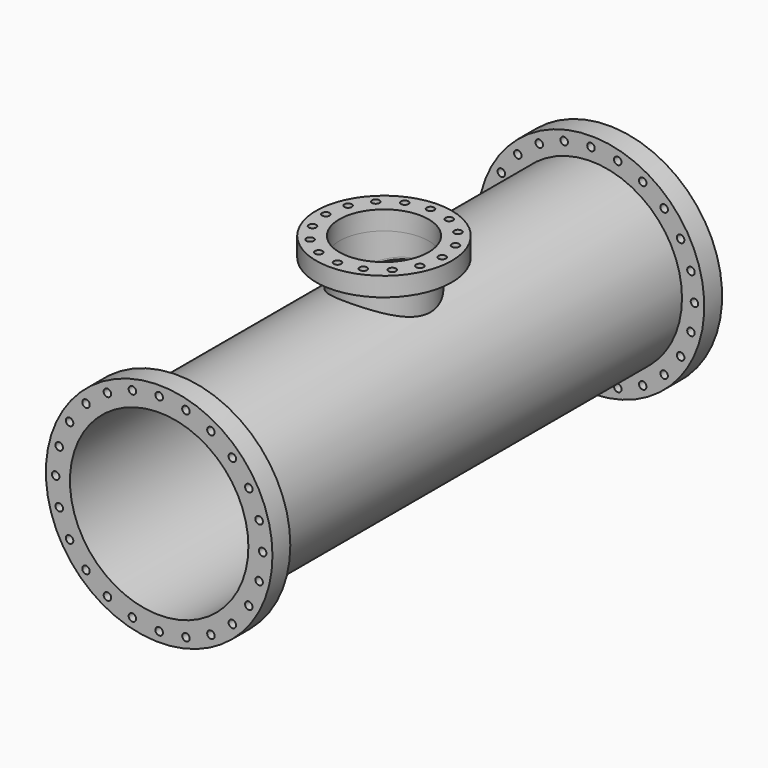
from build123d import *

# Parameters (mm, degrees)
F0_R      = 102
F0_R_2    = 100
F1_DEPTH  = 580
F2_R      = 127
F2_R_2    = 102
F2_R_3    = 100
F3_DEPTH  = 25
F4_R      = 127
F4_R_2    = 102
F4_R_3    = 100
F5_DEPTH  = 25
F7_D      = 8.4
F9_R      = 52
F9_R_2    = 50
F10_REACH = 399.0792104868
F11_REACH = 393.4223562373
F9_R_3    = 76
F12_DEPTH = 21.3
F14_D     = 8.4
F14_DEPTH = 27
F14_TIP   = 2.5236145999


with BuildPart() as f1:
    # F0 (on Front) → F1 (new body)
    with BuildSketch(Plane.XZ):
        Circle(F0_R)
        Circle(F0_R_2, mode=Mode.SUBTRACT)
    extrude(amount=F1_DEPTH)

    # F2 (on face) → F3 (join)
    with BuildSketch(Plane.XZ.offset(580)):
        Circle(F2_R)
        Circle(F2_R_2, mode=Mode.SUBTRACT)
        Circle(F2_R_2)
        Circle(F2_R_3, mode=Mode.SUBTRACT)
    extrude(amount=F3_DEPTH)

    # F4 (on face) → F5 (join)
    with BuildSketch(Plane(origin=(0, 0, 0), x_dir=(-1, 0, 0), z_dir=(0, 1, 0))):
        Circle(F4_R)
        Circle(F4_R_2, mode=Mode.SUBTRACT)
        Circle(F4_R_2)
        Circle(F4_R_3, mode=Mode.SUBTRACT)
    extrude(amount=F5_DEPTH)

    # F7 (through all)
    with Locations(Plane(origin=(0, 25, 0), x_dir=(-1, 0, 0), z_dir=(0, 1, 0))):
        with Locations((0, 116), (30.0230092319, 112.0473958495), (58, 100.458946839), (82.0243866176, 82.0243866176), (100.458946839, 58), (112.0473958495, 30.0230092319), (116, 0), (112.0473958495, -30.0230092319), (100.458946839, -58), (82.0243866176, -82.0243866176), (58, -100.458946839), (30.0230092319, -112.0473958495), (0, -116), (-30.0230092319, -112.0473958495), (-58, -100.458946839), (-82.0243866176, -82.0243866176), (-100.458946839, -58), (-112.0473958495, -30.0230092319), (-116, 0), (-112.0473958495, 30.0230092319), (-100.458946839, 58), (-82.0243866176, 82.0243866176), (-58, 100.458946839), (-30.0230092319, 112.0473958495)):
            Hole(F7_D / 2)

    f10_end = f1.faces().sort_by_distance((-102, -290, 0))[0]
    # F9 (on offset) → F10 (join, up to a face of the model that its end follows)
    with BuildSketch(Plane.XY.offset(125)):
        with Locations((0, -290)):
            Circle(F9_R)
        with Locations((0, -290)):
            Circle(F9_R_2, mode=Mode.SUBTRACT)
    f10_long = extrude(amount=-F10_REACH, mode=Mode.PRIVATE)
    add(split(f10_long, bisect_by=f10_end, keep=Keep.ALL, mode=Mode.PRIVATE).solids().sort_by_distance((-50.5292178951, -290, 125))[0])

    f11_end = f1.faces().sort_by_distance((-100, -302.5, 0))[0]
    # F9 (on offset) → F11 (cut, up to a face of the model that its end follows)
    with BuildSketch(Plane.XY.offset(125)):
        with Locations((0, -290)):
            Circle(F9_R_2)
    f11_long = extrude(amount=-F11_REACH, mode=Mode.PRIVATE)
    add(split(f11_long, bisect_by=f11_end, keep=Keep.ALL, mode=Mode.PRIVATE).solids().sort_by_distance((0, -290, 125))[0], mode=Mode.SUBTRACT)

    # F9 (on offset) → F12 (join)
    with BuildSketch(Plane.XY.offset(125)):
        with Locations((0, -290)):
            Circle(F9_R_3)
        with Locations((0, -290)):
            Circle(F9_R, mode=Mode.SUBTRACT)
        with Locations((0, -290)):
            Circle(F9_R)
        with Locations((0, -290)):
            Circle(F9_R_2, mode=Mode.SUBTRACT)
    extrude(amount=F12_DEPTH)

    # F14
    with Locations(Plane.XY.offset(146.3)):
        with Locations((0, -224.85), (24.9318256186, -229.8092484569), (46.0680067943, -243.9319932057), (60.1907515431, -265.0681743814), (65.15, -290), (60.1907515431, -314.9318256186), (46.0680067943, -336.0680067943), (24.9318256186, -350.1907515431), (0, -355.15), (-24.9318256186, -350.1907515431), (-46.0680067943, -336.0680067943), (-60.1907515431, -314.9318256186), (-65.15, -290), (-60.1907515431, -265.0681743814), (-46.0680067943, -243.9319932057), (-24.9318256186, -229.8092484569)):
            Hole(F14_D / 2, depth=F14_DEPTH)
            with Locations((0, 0, -(F14_DEPTH + F14_TIP / 2))):  # 118° drill point
                Cone(0, F14_D / 2, F14_TIP, mode=Mode.SUBTRACT)


solid = f1.part
